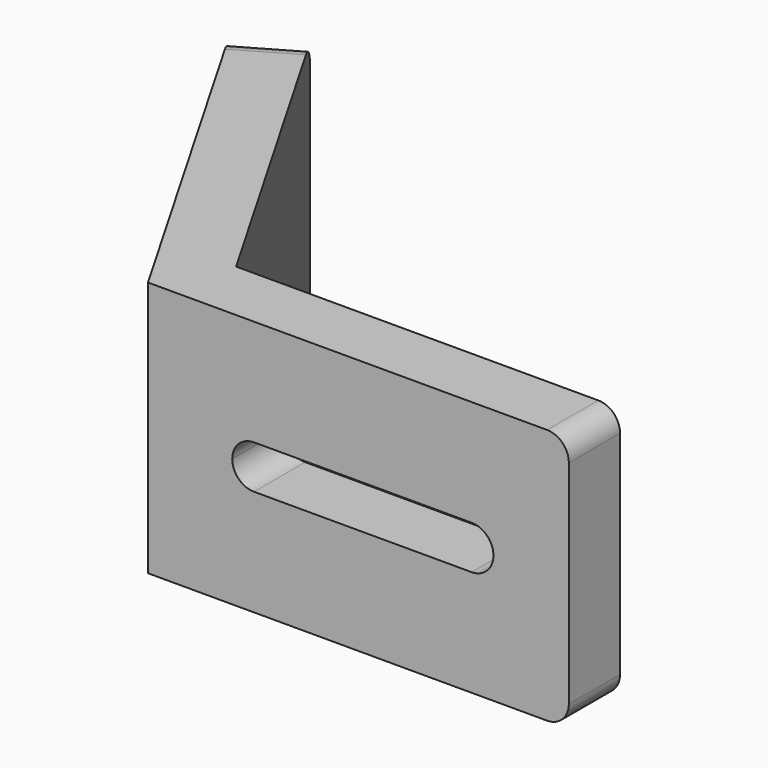
from build123d import *

# Parameters (mm, degrees)
F1_DEPTH = 20
F2_W     = 20.4075463116
F2_H     = 3.4
F3_DEPTH = 25
F4_R     = 1.69999


# Not quite as in the source:
# - a fillet or chamfer is up to 0.001 mm smaller than in the source, because OpenCascade refuses the exact size


with BuildPart() as f1:
    # F0 (on Top) → F1 (new body)
    with BuildSketch(Plane.XY):
        Polygon((-2.8867513459, 0), (0, 0), (30, 0), (30, 5), (0, 5), (-15, 30.9807621135), (-19.3301270189, 28.4807621135), align=None)
    extrude(amount=F1_DEPTH)

    # F2 (on face) → F3 (cut)
    with BuildSketch(Plane.XZ):
        with Locations((13.9012318105, 10)):
            Rectangle(F2_W, F2_H)
    extrude(amount=-F3_DEPTH, mode=Mode.SUBTRACT)

    # F4 (radius 1.7 in the source; OpenCascade refuses exactly that, so slightly less here)
    f4_edges = [f1.edges().sort_by_distance(p)[0] for p in [
        (3.697459, 2.5, 8.3),
        (3.697459, 2.5, 11.7),
        (24.105005, 2.5, 11.7),
        (24.105005, 2.5, 8.3),
        (30, 2.5, 20),
        (30, 2.5, 0),
        (-17.165064, 29.730762, 20),
        (-17.165064, 29.730762, 0),
    ]]
    fillet(f4_edges, radius=F4_R)


solid = f1.part
